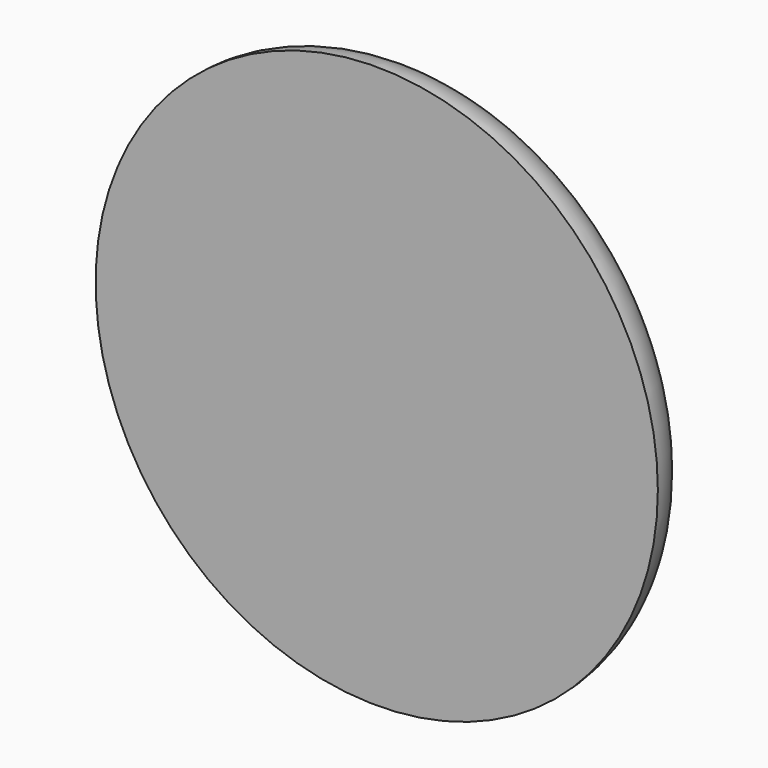
from build123d import *

# Parameters (mm, degrees)
F0_R         = 27.5
F1_DEPTH     = 5
F2_R         = 4.99999
F3_TEXT_SIZE = 39.881947709
F4_DEPTH     = 0.5


# Not quite as in the source:
# - a fillet or chamfer is up to 0.001 mm smaller than in the source, because OpenCascade refuses the exact size
# - Text() gives the source's letters only with a copy of the font that has no kerning and outlines rounded to 1/6400 em; it was checked with that copy


with BuildPart() as f1:
    # F0 (on Front) → F1 (new body)
    with BuildSketch(Plane.XZ):
        with Locations((-16.1759364117, 22.2393588308)):
            Circle(F0_R)
    extrude(amount=F1_DEPTH)

    # F2 (radius 5 in the source; OpenCascade refuses exactly that, so slightly less here)
    f2_edges = [f1.edges().sort_by_distance(p)[0] for p in [
        (-43.675936, 0, 22.239359),
    ]]
    fillet(f2_edges, radius=F2_R)

    # F3 (on face) → F4 (join)
    with BuildSketch(Plane(origin=(0, 0, 0), x_dir=(-1, 0, 0), z_dir=(0, 1, 0))):
        with Locations((4.9736378714, 7.5298035517)):
            Text('b', F3_TEXT_SIZE, font='Open Sans', font_style=FontStyle.BOLD, text_align=(TextAlign.LEFT, TextAlign.BOTTOM))
    extrude(amount=F4_DEPTH)


solid = f1.part
